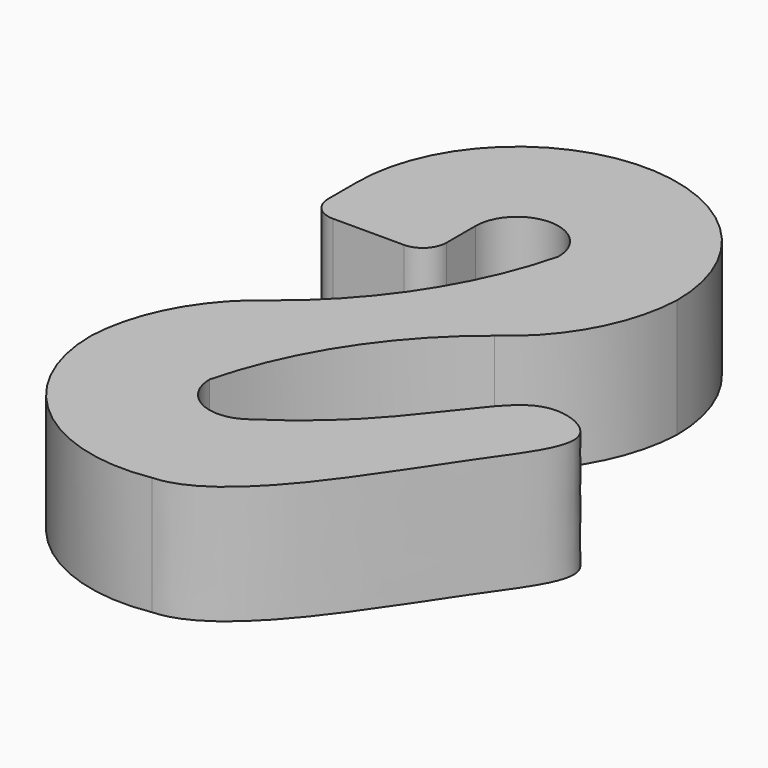
from build123d import *

# Parameters (mm, degrees)
F1_DEPTH = 5
F2_R     = 1


with BuildPart() as f1:
    # F0 (on Top) → F1 (new body)
    with BuildSketch(Plane.XY):
        with BuildLine():
            ThreePointArc((3.8771553396, 2.9075231471), (6.0924160212, 5.4090511435), (6.9899855634, 8.6276519452))
            ThreePointArc((6.9899855634, 8.6276519452), (0.2399855634, 15.3893333343), (-6.5100144366, 8.6276519452))
            Line((-6.5100144366, 8.6276519452), (-6.5100144366, 6.0996299018))
            Line((-6.5100144366, 6.0996299018), (-1.5100144366, 6.0996299018))
            Line((-1.5100144366, 6.0996299018), (-1.5100144366, 8.6276519452))
            ThreePointArc((-1.5100144366, 8.6276519452), (0.2399855634, 10.3776519452), (1.9899855634, 8.6276519452))
            ThreePointArc((1.9899855634, 8.6276519452), (-0.0176334179, 4.0282165309), (-3.3971842127, 0.3182331711))
            ThreePointArc((-3.3971842127, 0.3182331711), (-5.6124448943, -2.1832948252), (-6.5100144366, -5.4018956269))
            ThreePointArc((-6.5100144366, -5.4018956269), (-4.1110010202, -10.5741436346), (1.3922955876, -12.0644930136))
            add(Edge.make_bspline(
                [(1.3922955876, -12.0644930136), (-0.1266799353, -12.1261417215), (-3.3351189393, -9.5714125443), (-0.1444645506, -7.7520643513), (1.1719607323, -6.8830851099)],
                knots=[0.7707273739, 0.7707273739, 0.7707273739, 0.7707273739, 0.8831647339, 0.9980209114, 0.9980209114, 0.9980209114, 0.9980209114], degree=3))
            ThreePointArc((1.1719607323, -6.8830851099), (-0.6060473716, -6.9337991072), (-1.5100144366, -5.4018956269))
            ThreePointArc((-1.5100144366, -5.4018956269), (0.4976045447, -0.8024602126), (3.8771553396, 2.9075231471))
        make_face()
        with BuildLine():
            ThreePointArc((1.2397373462, -6.838209093), (1.2061096332, -6.8610406786), (1.1719607323, -6.8830851099))
            add(Edge.make_bspline(
                [(1.3922955876, -12.0644930136), (-0.1266799353, -12.1261417215), (-3.3351189393, -9.5714125443), (-0.1444645506, -7.7520643513), (1.1719607323, -6.8830851099)],
                knots=[0.7707273739, 0.7707273739, 0.7707273739, 0.7707273739, 0.8831647339, 0.9980209114, 0.9980209114, 0.9980209114, 0.9980209114], degree=3))
            add(Edge.make_bspline(
                [(1.2397373462, -6.838209093), (2.5681971331, -5.9557774363), (4.4723284438, -4.3504476654), (6.6235674258, -1.4102036415), (8.3753207128, 0.4943501627), (11.5028973428, -0.8405099917), (8.8134499394, -4.3647410583), (6.8147363685, -7.6666050922), (3.3824715958, -11.9837202971), (1.3922955876, -12.0644930136)],
                knots=[0, 0, 0, 0, 0.1168622127, 0.2252853805, 0.3125926323, 0.3959885324, 0.5007919029, 0.623410888, 0.7707273739, 0.7707273739, 0.7707273739, 0.7707273739], degree=3))
        make_face()
    extrude(amount=F1_DEPTH)

    # F2
    f2_edges = [f1.edges().sort_by_distance(p)[0] for p in [
        (-1.510014, 6.09963, 2.5),
        (-6.510014, 6.09963, 2.5),
    ]]
    fillet(f2_edges, radius=F2_R)


solid = f1.part
